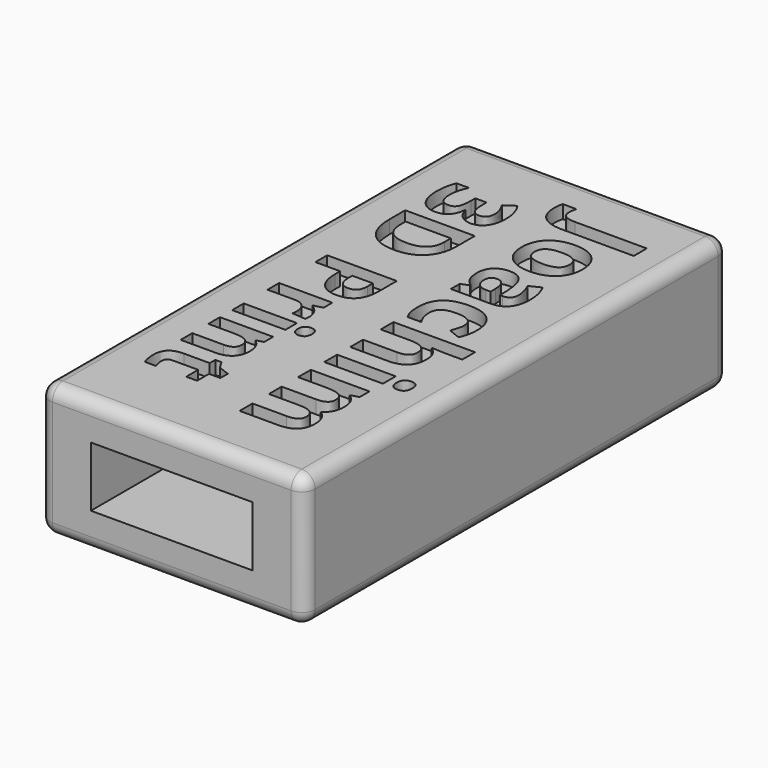
from build123d import *

# Parameters (mm, degrees)
F0_W         = 20
F0_H         = 10
F2_DEPTH     = 40
F1_W         = 12.2
F1_H         = 4.53
F3_DEPTH     = 25
F4_R         = 1
F5_TEXT_SIZE = 8.09381467
F6_DEPTH     = 1
F7_TEXT_SIZE = 7.3492822967
F8_DEPTH     = 1


# Not quite as in the source:
# - Text() gives the source's letters only with a copy of the font that has no kerning and outlines rounded to 1/6400 em; it was checked with that copy


with BuildPart() as f2:
    # F0 (on Front) → F2 (new body)
    with BuildSketch(Plane.XZ):
        Rectangle(F0_W, F0_H)
    extrude(amount=-F2_DEPTH)

    # F1 (on Front) → F3 (cut)
    with BuildSketch(Plane.XZ):
        Rectangle(F1_W, F1_H)
    extrude(amount=-F3_DEPTH, mode=Mode.SUBTRACT)

    # F4
    f4_edges = [f2.edges().sort_by_distance(p)[0] for p in [
        (10, 20, 5),
        (0, 40, 5),
        (-10, 20, 5),
        (-10, 20, -5),
        (-10, 40, 0),
        (0, 0, -5),
        (0, 0, 5),
        (10, 0, 0),
        (10, 20, -5),
        (0, 40, -5),
        (10, 40, 0),
        (-10, 0, 0),
    ]]
    fillet(f4_edges, radius=F4_R)

    # F5 (on face) → F6 (cut)
    with BuildSketch(Plane.XY.offset(5)):
        with Locations(Location((1.5027987204, 36.3898171542), (0, 0, -90))):
            Text('Joachim', F5_TEXT_SIZE, font='Open Sans', font_style=FontStyle.BOLD, text_align=(TextAlign.LEFT, TextAlign.BOTTOM))
    extrude(amount=-F6_DEPTH, mode=Mode.SUBTRACT)

    # F7 (on face) → F8 (cut)
    with BuildSketch(Plane.XY.offset(5)):
        with Locations(Location((-6.8657157214, 35.4335972836), (0, 0, -90))):
            Text('3D Print', F7_TEXT_SIZE, font='Open Sans', font_style=FontStyle.BOLD, text_align=(TextAlign.LEFT, TextAlign.BOTTOM))
    extrude(amount=-F8_DEPTH, mode=Mode.SUBTRACT)


solid = f2.part
